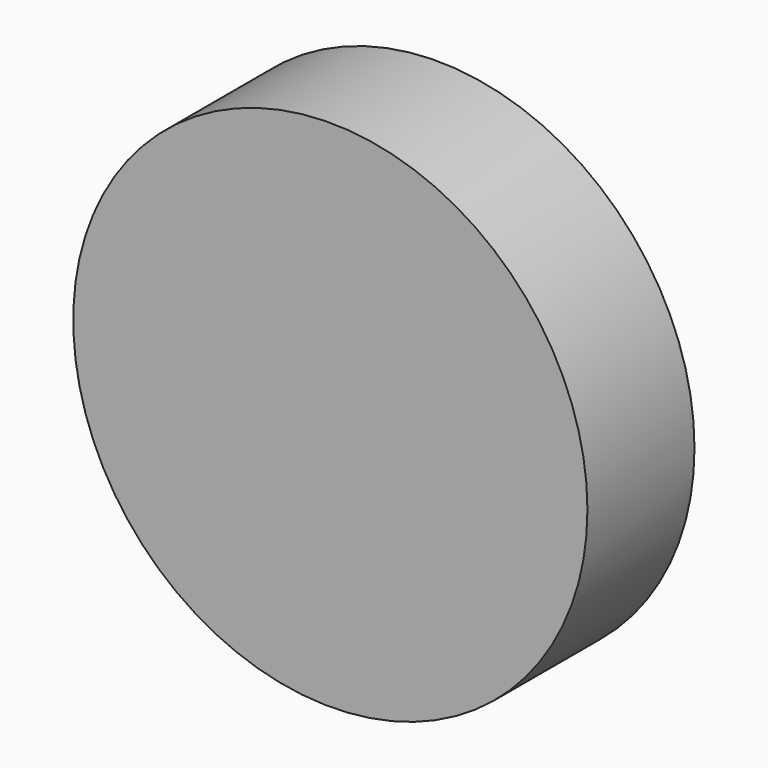
from build123d import *

# Parameters (mm, degrees)
F0_R     = 48.7885127136
F1_DEPTH = 25.4


# Not quite as in the source:
# - the program builds the solid bodies; features that only make, move or delete a surface that nothing else refers to are left out


with BuildPart() as f1:
    # F0 (on Front) → F1 (new body)
    with BuildSketch(Plane.XZ):
        with Locations((-3.7921343464, 0)):
            Circle(F0_R)
    extrude(amount=F1_DEPTH)


solid = f1.part
